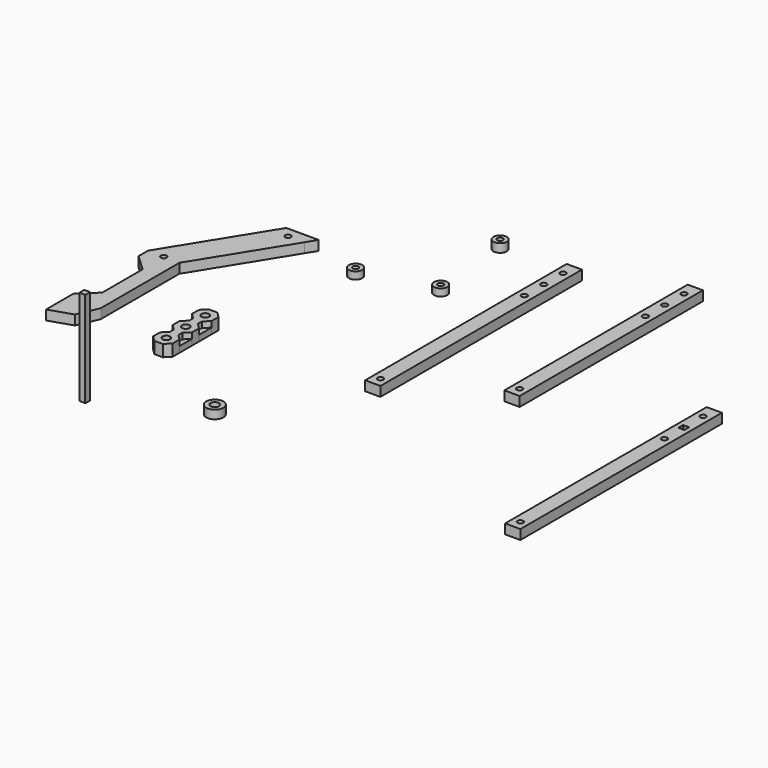
from build123d import *

# Parameters (mm, degrees)
F1_DEPTH  = 5.08
F0_W      = 8
F0_H      = 117
F0_H_2    = 15
F0_R      = 1.5
F0_H_3    = 105
F0_W_2    = 3.15
F0_H_4    = 3.15
F2_DEPTH  = 50
F0_R_2    = 3.5
F3_DEPTH  = 4.45
F0_R_3    = 4.5
F0_R_4    = 2.25
F4_R      = 0.25
F5_R      = 3.5
F5_R_2    = 1.5
F6_DEPTH  = 3.815
F8_DEPTH  = 3.1
F7_W      = 2.25
F7_H      = 2.55
F9_DEPTH  = 6.15
F10_DEPTH = 3.764


# Not quite as in the source:
# - a feature names something its author has since deleted; it is built from what else it names


with BuildPart() as f1:
    # F0 (on Top) → F1 (new body)
    with BuildSketch(Plane.XY):
        with BuildLine():
            Line((-50.949690631, 43.8997100926), (-67.949690631, 43.8997100926))
            Line((-67.949690631, 43.8997100926), (-71.2368406563, 38.5939453388))
            Line((-71.2368406563, 38.5939453388), (-64.2368406563, 38.5939453388))
            ThreePointArc((-64.2368406563, 38.5939453388), (-62.7368406563, 40.0939453388), (-61.2368406563, 38.5939453388))
            Line((-61.2368406563, 38.5939453388), (-54.2368406563, 38.5939453388))
            Line((-54.2368406563, 38.5939453388), (-50.949690631, 43.8997100926))
        make_face()
        Polygon((-90.9492363239, -13.4048849161), (-99.5492363239, -13.4048849161), (-90.9492363239, -21.4048934984), align=None)
        Polygon((-90.9492363239, -55.9028989029), (-90.9492363239, -47.8827440429), (-99.5708935492, -55.9028989029), align=None)
        with BuildLine():
            Line((-64.2368406563, 38.5939453388), (-71.2368406563, 38.5939453388))
            Line((-71.2368406563, 38.5939453388), (-99.5492363239, -7.1048849161))
            Line((-99.5492363239, -7.1048849161), (-92.680417628, -7.2793228948))
            ThreePointArc((-92.680417628, -7.2793228948), (-91.1618589797, -5.8175249342), (-89.6809010977, -7.3174040619))
            ThreePointArc((-89.6809010977, -7.3174040619), (-89.6810219699, -7.3364461799), (-89.6813845673, -7.3554852291))
            Line((-89.6813845673, -7.3554852291), (-82.8125658714, -7.5299232078))
            Line((-82.8125658714, -7.5299232078), (-54.2368406563, 38.5939453388))
            Line((-54.2368406563, 38.5939453388), (-61.2368406563, 38.5939453388))
            ThreePointArc((-61.2368406563, 38.5939453388), (-62.7368406563, 37.0939453388), (-64.2368406563, 38.5939453388))
        make_face()
        with BuildLine():
            Line((-92.680417628, -7.2793228948), (-99.5492363239, -7.1048849161))
            Line((-99.5492363239, -7.1048849161), (-99.5492363239, -13.4048849161))
            Line((-99.5492363239, -13.4048849161), (-90.9492363239, -13.4048849161))
            Line((-90.9492363239, -13.4048849161), (-90.9492363239, -21.4048934984))
            Line((-90.9492363239, -21.4048934984), (-90.9492363239, -47.8827440429))
            Line((-90.9492363239, -47.8827440429), (-90.9492363239, -55.9028989029))
            Line((-90.9492363239, -55.9028989029), (-99.5708935492, -55.9028989029))
            Line((-99.5708935492, -55.9028989029), (-99.5708935492, -73.9028989029))
            Line((-99.5708935492, -73.9028989029), (-87.5764183456, -70.0438103329))
            Line((-87.5764183456, -70.0438103329), (-82.8125658714, -59.0299232078))
            Line((-82.8125658714, -59.0299232078), (-82.8125658714, -7.5299232078))
            Line((-82.8125658714, -7.5299232078), (-89.6813845673, -7.3554852291))
            ThreePointArc((-89.6813845673, -7.3554852291), (-91.2189822648, -8.8169205923), (-92.680417628, -7.2793228948))
        make_face()
    extrude(amount=F1_DEPTH)


with BuildPart() as f1b:
    # F0 (on Top) → F1, piece 2 (new body)
    with BuildSketch(Plane.XY):
        with Locations((45.5790795386, 17.1512553096)):
            Rectangle(F0_W, F0_H)
        with BuildLine():
            ThreePointArc((47.0790795386, -36.3287446904), (44.5184193668, -37.3894048622), (45.5790795386, -34.8287446904))
            ThreePointArc((45.5790795386, -34.8287446904), (46.6397397104, -35.2680845186), (47.0790795386, -36.3287446904))
        make_face(mode=Mode.SUBTRACT)
        with BuildLine():
            ThreePointArc((45.5790795386, 56.4312553096), (44.0790795386, 57.9312553096), (45.5790795386, 59.4312553096))
            ThreePointArc((45.5790795386, 59.4312553096), (46.6397397104, 58.9919154814), (47.0790795386, 57.9312553096))
            ThreePointArc((47.0790795386, 57.9312553096), (46.6397397104, 56.8705951378), (45.5790795386, 56.4312553096))
        make_face(mode=Mode.SUBTRACT)
        with BuildLine():
            ThreePointArc((47.0790795386, 70.6312553096), (46.6397397104, 69.5705951378), (45.5790795386, 69.1312553096))
            ThreePointArc((45.5790795386, 69.1312553096), (44.5184193668, 71.6919154814), (47.0790795386, 70.6312553096))
        make_face(mode=Mode.SUBTRACT)
        with Locations((45.5790795386, 83.1512553096)):
            Rectangle(F0_W, F0_H_2)
        with Locations((45.5790795386, 83.3312553096)):
            Circle(F0_R, mode=Mode.SUBTRACT)
    extrude(amount=F1_DEPTH)


with BuildPart() as f1c:
    # F0 (on Top) → F1, piece 3 (new body)
    with BuildSketch(Plane.XY):
        with Locations((95.6552401185, 39.7728151456)):
            Rectangle(F0_W, F0_H_3)
        with BuildLine():
            ThreePointArc((97.1552401185, -7.7271848544), (94.5945799467, -8.7878450262), (95.6552401185, -6.2271848544))
            ThreePointArc((95.6552401185, -6.2271848544), (96.7159002903, -6.6665246827), (97.1552401185, -7.7271848544))
        make_face(mode=Mode.SUBTRACT)
        with BuildLine():
            ThreePointArc((95.6552401185, 73.0728151456), (94.1552401185, 74.5728151456), (95.6552401185, 76.0728151456))
            ThreePointArc((95.6552401185, 76.0728151456), (96.7159002903, 75.6334753173), (97.1552401185, 74.5728151456))
            ThreePointArc((97.1552401185, 74.5728151456), (96.7159002903, 73.5121549738), (95.6552401185, 73.0728151456))
        make_face(mode=Mode.SUBTRACT)
        with BuildLine():
            ThreePointArc((97.1552401185, 87.2728151456), (96.7159002903, 86.2121549738), (95.6552401185, 85.7728151456))
            ThreePointArc((95.6552401185, 85.7728151456), (94.5945799467, 88.3334753173), (97.1552401185, 87.2728151456))
        make_face(mode=Mode.SUBTRACT)
        with Locations((95.6552401185, 99.7728151456)):
            Rectangle(F0_W, F0_H_2)
        with Locations((95.6552401185, 99.9728151456)):
            Circle(F0_R, mode=Mode.SUBTRACT)
    extrude(amount=F1_DEPTH)


with BuildPart() as f1d:
    # F0 (on Top) → F1, piece 4 (new body)
    with BuildSketch(Plane.XY):
        with Locations((169.5275753736, -46.1102230102)):
            Rectangle(F0_W, F0_H)
        with BuildLine():
            ThreePointArc((171.0275753736, -99.6102230102), (168.4669152019, -100.670883182), (169.5275753736, -98.1102230102))
            ThreePointArc((169.5275753736, -98.1102230102), (170.5882355454, -98.5495628384), (171.0275753736, -99.6102230102))
        make_face(mode=Mode.SUBTRACT)
        with BuildLine():
            ThreePointArc((171.0275753736, -5.3102230102), (170.5882355454, -6.370883182), (169.5275753736, -6.8102230102))
            ThreePointArc((169.5275753736, -6.8102230102), (168.0275753736, -5.3102230102), (169.5275753736, -3.8102230102))
            ThreePointArc((169.5275753736, -3.8102230102), (170.5882355454, -4.2495628384), (171.0275753736, -5.3102230102))
        make_face(mode=Mode.SUBTRACT)
        with BuildLine():
            ThreePointArc((170.8877224245, 5.7897769898), (170.252144211, 5.4187366554), (169.5275753736, 5.2897769898))
            ThreePointArc((169.5275753736, 5.2897769898), (168.8030065363, 5.4187366554), (168.1674283228, 5.7897769898))
            Line((168.1674283228, 5.7897769898), (167.9275753736, 5.7897769898))
            Line((167.9275753736, 5.7897769898), (167.9275753736, 6.0296299389))
            ThreePointArc((167.9275753736, 6.0296299389), (167.4275753736, 7.3897769898), (167.9275753736, 8.7499240407))
            Line((167.9275753736, 8.7499240407), (167.9275753736, 8.9897769898))
            Line((167.9275753736, 8.9897769898), (168.1674283228, 8.9897769898))
            ThreePointArc((168.1674283228, 8.9897769898), (169.5275753736, 9.4897769898), (170.8877224245, 8.9897769898))
            Line((170.8877224245, 8.9897769898), (171.1275753736, 8.9897769898))
            Line((171.1275753736, 8.9897769898), (171.1275753736, 8.7499240407))
            ThreePointArc((171.1275753736, 8.7499240407), (171.4986157081, 8.1143458271), (171.6275753736, 7.3897769898))
            ThreePointArc((171.6275753736, 7.3897769898), (171.4986157081, 6.6652081525), (171.1275753736, 6.0296299389))
            Line((171.1275753736, 6.0296299389), (171.1275753736, 5.7897769898))
            Line((171.1275753736, 5.7897769898), (170.8877224245, 5.7897769898))
        make_face(mode=Mode.SUBTRACT)
        with Locations((169.5275753736, 19.8897769898)):
            Rectangle(F0_W, F0_H_2)
        with Locations((169.5275753736, 20.0897769898)):
            Circle(F0_R, mode=Mode.SUBTRACT)
        with BuildLine():
            ThreePointArc((170.8877224245, 8.9897769898), (169.5275753736, 9.4897769898), (168.1674283228, 8.9897769898))
            Line((168.1674283228, 8.9897769898), (170.8877224245, 8.9897769898))
        make_face()
        with BuildLine():
            ThreePointArc((167.9275753736, 8.7499240407), (167.4275753736, 7.3897769898), (167.9275753736, 6.0296299389))
            Line((167.9275753736, 6.0296299389), (167.9275753736, 8.7499240407))
        make_face()
        with BuildLine():
            Line((171.1275753736, 8.7499240407), (171.1275753736, 6.0296299389))
            ThreePointArc((171.1275753736, 6.0296299389), (171.4986157081, 6.6652081525), (171.6275753736, 7.3897769898))
            ThreePointArc((171.6275753736, 7.3897769898), (171.4986157081, 8.1143458271), (171.1275753736, 8.7499240407))
        make_face()
        with BuildLine():
            Line((169.5275753736, 5.7897769898), (169.5275753736, 5.2897769898))
            ThreePointArc((169.5275753736, 5.2897769898), (170.252144211, 5.4187366554), (170.8877224245, 5.7897769898))
            Line((170.8877224245, 5.7897769898), (169.5275753736, 5.7897769898))
        make_face()
        with BuildLine():
            ThreePointArc((168.1674283228, 5.7897769898), (168.8030065363, 5.4187366554), (169.5275753736, 5.2897769898))
            Line((169.5275753736, 5.2897769898), (169.5275753736, 5.7897769898))
            Line((169.5275753736, 5.7897769898), (168.1674283228, 5.7897769898))
        make_face()
        with BuildLine():
            ThreePointArc((170.8877224245, 8.9897769898), (171.0124996141, 8.8747012303), (171.1275753736, 8.7499240407))
            Line((171.1275753736, 8.7499240407), (171.1275753736, 8.9897769898))
            Line((171.1275753736, 8.9897769898), (170.8877224245, 8.9897769898))
        make_face()
        with BuildLine():
            Line((167.9275753736, 8.9897769898), (167.9275753736, 8.7499240407))
            ThreePointArc((167.9275753736, 8.7499240407), (168.0426511332, 8.8747012303), (168.1674283228, 8.9897769898))
            Line((168.1674283228, 8.9897769898), (167.9275753736, 8.9897769898))
        make_face()
        with BuildLine():
            Line((167.9275753736, 5.7897769898), (168.1674283228, 5.7897769898))
            ThreePointArc((168.1674283228, 5.7897769898), (168.0426511332, 5.9048527493), (167.9275753736, 6.0296299389))
            Line((167.9275753736, 6.0296299389), (167.9275753736, 5.7897769898))
        make_face()
        with BuildLine():
            ThreePointArc((171.1275753736, 6.0296299389), (171.0124996141, 5.9048527493), (170.8877224245, 5.7897769898))
            Line((170.8877224245, 5.7897769898), (171.1275753736, 5.7897769898))
            Line((171.1275753736, 5.7897769898), (171.1275753736, 6.0296299389))
        make_face()
    extrude(amount=F1_DEPTH)


with BuildPart() as f2:
    # F0 (on Top) → F2 (new body)
    with BuildSketch(Plane.XY):
        with Locations((-42.7516108632, -119.568117547)):
            Rectangle(F0_W_2, F0_H_4)
        with Locations((-42.7516108632, -119.568117547)):
            Circle(F0_R, mode=Mode.SUBTRACT)
        with Locations((-42.7516108632, -119.568117547)):
            Circle(F0_R)
    extrude(amount=F2_DEPTH)

    # F4
    f4_edges = [f2.edges().sort_by_distance(p)[0] for p in [
        (-41.176611, -121.143118, 25),
        (-44.326611, -117.993118, 25),
        (-44.326611, -121.143118, 25),
        (-41.176611, -117.993118, 25),
    ]]
    fillet(f4_edges, radius=F4_R)


with BuildPart() as f3:
    # F0 (on Top) → F3 (new body)
    with BuildSketch(Plane.XY):
        with Locations((5.9054424055, 91.6430652142)):
            Circle(F0_R_2)
        with Locations((5.9054424055, 91.6430652142)):
            Circle(F0_R, mode=Mode.SUBTRACT)
    extrude(amount=F3_DEPTH)


with BuildPart() as f3b:
    # F0 (on Top) → F3, piece 2 (new body)
    with BuildSketch(Plane.XY):
        with Locations((6.2566562556, -95.6798642874)):
            Circle(F0_R_3)
        with Locations((6.2566562556, -95.6798642874)):
            Circle(F0_R_4, mode=Mode.SUBTRACT)
    extrude(amount=F3_DEPTH)


with BuildPart() as f6:
    # F5 (on Top) → F6 (new body)
    with BuildSketch(Plane.XY):
        with Locations((-25.4324208945, 36.1619368196)):
            Circle(F5_R)
        with Locations((-25.4324208945, 36.1619368196)):
            Circle(F5_R_2, mode=Mode.SUBTRACT)
    extrude(amount=F6_DEPTH)


with BuildPart() as f8:
    # F7 (on Top) → F8 (new body)
    with BuildSketch(Plane.XY):
        Polygon((-39.0240414023, -49.4567692398), (-39.0240414023, -41.1911208631), (-41.8740414023, -44.0489450514), (-41.8740414023, -46.5989450514), align=None)
    extrude(amount=F8_DEPTH)


with BuildPart() as f8b:
    # F7 (on Top) → F8, piece 2 (new body)
    with BuildSketch(Plane.XY):
        Polygon((-46.3740414023, -46.5989450514), (-46.3740414023, -44.0489450514), (-49.2240414023, -41.1911208631), (-49.2240414023, -49.4567692398), align=None)
    extrude(amount=F8_DEPTH)


with BuildPart() as f8c:
    # F7 (on Top) → F8, piece 3 (new body)
    with BuildSketch(Plane.XY):
        Polygon((-46.3740414023, -56.7989450514), (-49.2240414023, -53.9567692398), (-49.2240414023, -62.1911208631), (-46.3740414023, -59.3489450514), align=None)
    extrude(amount=F8_DEPTH)


with BuildPart() as f8d:
    # F7 (on Top) → F8, piece 4 (new body)
    with BuildSketch(Plane.XY):
        Polygon((-39.0240414023, -62.1911208631), (-39.0240414023, -53.9567692398), (-41.8740414023, -56.7989450514), (-41.8740414023, -59.3489450514), align=None)
    extrude(amount=F8_DEPTH)


with BuildPart() as f9:
    # F7 (on Top) → F9 (new body)
    with BuildSketch(Plane.XY):
        with BuildLine():
            ThreePointArc((-44.1240414023, -40.9489450514), (-45.5382549647, -37.5347314891), (-42.1240414023, -38.9489450514))
            Line((-42.1240414023, -38.9489450514), (-39.0240414023, -38.9489450514))
            Line((-39.0240414023, -38.9489450514), (-39.0240414023, -36.6911208631))
            Line((-39.0240414023, -36.6911208631), (-41.8740414023, -33.8489450514))
            Line((-41.8740414023, -33.8489450514), (-46.3740414023, -33.8489450514))
            Line((-46.3740414023, -33.8489450514), (-49.2240414023, -36.6911208631))
            Line((-49.2240414023, -36.6911208631), (-49.2240414023, -41.1911208631))
            Line((-49.2240414023, -41.1911208631), (-46.3740414023, -44.0489450514))
            Line((-46.3740414023, -44.0489450514), (-44.1240414023, -44.0489450514))
            Line((-44.1240414023, -44.0489450514), (-44.1240414023, -40.9489450514))
        make_face()
        with BuildLine():
            Line((-39.0240414023, -38.9489450514), (-42.1240414023, -38.9489450514))
            ThreePointArc((-42.1240414023, -38.9489450514), (-42.70982784, -40.3631586138), (-44.1240414023, -40.9489450514))
            Line((-44.1240414023, -40.9489450514), (-44.1240414023, -44.0489450514))
            Line((-44.1240414023, -44.0489450514), (-41.8740414023, -44.0489450514))
            Line((-41.8740414023, -44.0489450514), (-39.0240414023, -41.1911208631))
            Line((-39.0240414023, -41.1911208631), (-39.0240414023, -38.9489450514))
        make_face()
        with BuildLine():
            Line((-41.8740414023, -46.5989450514), (-44.1240414023, -46.5989450514))
            Line((-44.1240414023, -46.5989450514), (-44.1240414023, -49.6989450514))
            ThreePointArc((-44.1240414023, -49.6989450514), (-42.70982784, -50.2847314891), (-42.1240414023, -51.6989450514))
            ThreePointArc((-42.1240414023, -51.6989450514), (-42.70982784, -53.1131586138), (-44.1240414023, -53.6989450514))
            Line((-44.1240414023, -53.6989450514), (-44.1240414023, -56.7989450514))
            Line((-44.1240414023, -56.7989450514), (-41.8740414023, -56.7989450514))
            Line((-41.8740414023, -56.7989450514), (-39.0240414023, -53.9567692398))
            Line((-39.0240414023, -53.9567692398), (-39.0240414023, -49.4567692398))
            Line((-39.0240414023, -49.4567692398), (-41.8740414023, -46.5989450514))
        make_face()
        with BuildLine():
            Line((-44.1240414023, -49.6989450514), (-44.1240414023, -46.5989450514))
            Line((-44.1240414023, -46.5989450514), (-46.3740414023, -46.5989450514))
            Line((-46.3740414023, -46.5989450514), (-49.2240414023, -49.4567692398))
            Line((-49.2240414023, -49.4567692398), (-49.2240414023, -53.9567692398))
            Line((-49.2240414023, -53.9567692398), (-46.3740414023, -56.7989450514))
            Line((-46.3740414023, -56.7989450514), (-44.1240414023, -56.7989450514))
            Line((-44.1240414023, -56.7989450514), (-44.1240414023, -53.6989450514))
            ThreePointArc((-44.1240414023, -53.6989450514), (-46.1240414023, -51.6989450514), (-44.1240414023, -49.6989450514))
        make_face()
        Polygon((-39.0240414023, -66.6911208631), (-39.0240414023, -62.1911208631), (-41.8740414023, -59.3489450514), (-44.1240414023, -59.3489450514), (-46.3740414023, -59.3489450514), (-49.2240414023, -62.1911208631), (-49.2240414023, -66.6911208631), (-46.3740414023, -69.5489450514), (-41.8740414023, -69.5489450514), align=None)
        with BuildLine():
            ThreePointArc((-42.1240414023, -64.4489450514), (-45.5382549647, -65.8631586138), (-44.1240414023, -62.4489450514))
            ThreePointArc((-44.1240414023, -62.4489450514), (-42.70982784, -63.0347314891), (-42.1240414023, -64.4489450514))
        make_face(mode=Mode.SUBTRACT)
        with Locations((-45.2490414023, -45.3239450514)):
            Rectangle(F7_W, F7_H)
        with Locations((-42.9990414023, -45.3239450514)):
            Rectangle(F7_W, F7_H)
        with Locations((-45.2490414023, -58.0739450514)):
            Rectangle(F7_W, F7_H)
        with Locations((-42.9990414023, -58.0739450514)):
            Rectangle(F7_W, F7_H)
    extrude(amount=F9_DEPTH)


with BuildPart() as f10:
    # F5 (on Top) → F10 (new body)
    with BuildSketch(Plane.XY):
        with Locations((11.1080519855, 46.2102368474)):
            Circle(F5_R)
        with Locations((11.1080519855, 46.2102368474)):
            Circle(F5_R_2, mode=Mode.SUBTRACT)
    extrude(amount=F10_DEPTH)


solid = Compound([f1.part, f1b.part, f1c.part, f1d.part, f2.part, f3.part, f3b.part, f6.part, f8.part, f8b.part, f8c.part, f8d.part, f9.part, f10.part])
